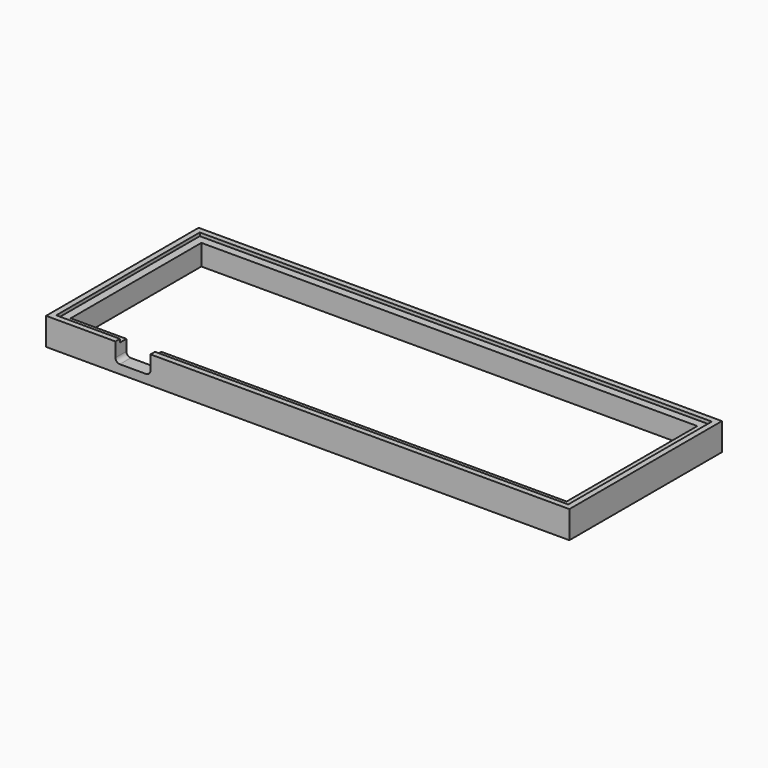
from build123d import *

# Parameters (mm, degrees)
F0_W     = 239.15
F0_H     = 87.15
F0_W_2   = 234
F0_H_2   = 82
F0_W_3   = 233
F0_H_3   = 81
F0_W_4   = 226.65
F0_H_4   = 74.65
F1_DEPTH = 12.525
F2_W     = 234
F2_H     = 82
F2_W_2   = 233
F2_H_2   = 81
F2_W_3   = 226.65
F2_H_3   = 74.65
F3_DEPTH = 1.5
F4_W     = 234
F4_H     = 82
F4_W_2   = 233
F4_H_2   = 81
F4_W_3   = 226.65
F4_H_3   = 74.65
F5_DEPTH = 1.5
F6_W     = 16
F6_H     = 9
F7_DEPTH = 10
F8_R     = 2


# Not quite as in the source:
# - a pattern or mirror of a feature is missing from the dataset's text; its kind, count and spacing are read off the source's solid


with BuildPart() as f1:
    # F0 (on Top) → F1 (new body)
    with BuildSketch(Plane.XY):
        Rectangle(F0_W, F0_H)
        Rectangle(F0_W_2, F0_H_2, mode=Mode.SUBTRACT)
        Rectangle(F0_W_2, F0_H_2)
        Rectangle(F0_W_3, F0_H_3, mode=Mode.SUBTRACT)
        Rectangle(F0_W_3, F0_H_3)
        Rectangle(F0_W_4, F0_H_4, mode=Mode.SUBTRACT)
    extrude(amount=F1_DEPTH)

    # F2 (on face) → F3 (cut)
    with BuildSketch(Plane.XY.offset(12.525)):
        Rectangle(F2_W, F2_H)
        Rectangle(F2_W_2, F2_H_2, mode=Mode.SUBTRACT)
        Rectangle(F2_W_2, F2_H_2)
        Rectangle(F2_W_3, F2_H_3, mode=Mode.SUBTRACT)
    f3 = extrude(amount=-F3_DEPTH, mode=Mode.SUBTRACT)

    # F3_copies: F3 across plane
    add(f3.mirror(Plane(origin=(0, 0, 6.2625), x_dir=(-1, 0, 0), z_dir=(0, 0, -1))), mode=Mode.SUBTRACT)

    # F4 (on face) → F5 (cut)
    with BuildSketch(Plane.XY):
        Rectangle(F4_W, F4_H)
        Rectangle(F4_W_2, F4_H_2, mode=Mode.SUBTRACT)
        Rectangle(F4_W_2, F4_H_2)
        Rectangle(F4_W_3, F4_H_3, mode=Mode.SUBTRACT)
    extrude(amount=-F5_DEPTH, mode=Mode.SUBTRACT)

    # F6 (on face) → F7 (cut)
    with BuildSketch(Plane.XZ.offset(43.575)):
        with Locations((-79.875, 8.5)):
            Rectangle(F6_W, F6_H)
    extrude(amount=-F7_DEPTH, mode=Mode.SUBTRACT)

    # F8
    f8_edges = [f1.edges().sort_by_distance(p)[0] for p in [
        (-71.875, -40.45, 4),
        (-87.875, -40.45, 4),
    ]]
    fillet(f8_edges, radius=F8_R)


solid = f1.part
